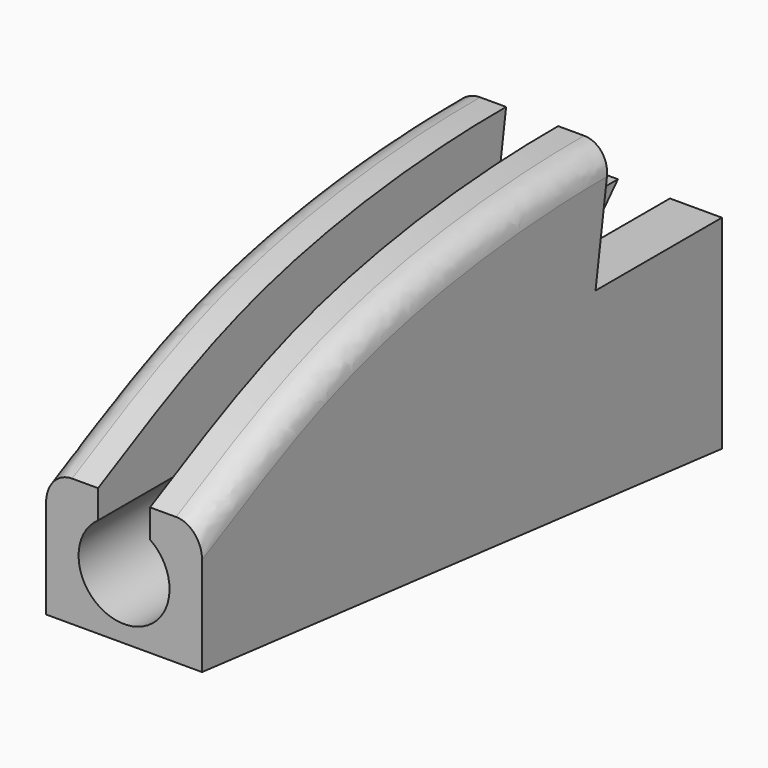
from build123d import *

# Parameters (mm, degrees)
F0_W           = 12
F0_H           = 50
F1_DEPTH       = 30
F3_D           = 7
F3_CSINK_D     = 12
F3_CSINK_ANGLE = 90
F4_W           = 4
F4_H           = 17.1277186767
F5_DEPTH       = 50
F11_DEPTH      = 12.5
F12_R          = 2
F15_DEPTH      = 12.5


# Not quite as in the source:
# - two fillets or chamfers of one size are made in one step
# - the dataset's text gives a spline's control points without its knots; the knots are read off the source's solid


with BuildPart() as f1:
    # F0 (on Top) → F1 (new body)
    with BuildSketch(Plane.XY):
        with Locations((0, -25)):
            Rectangle(F0_W, F0_H)
    extrude(amount=F1_DEPTH)

    # F3 (through all)
    with Locations(Plane(origin=(0, 0, 0), x_dir=(1, 0, 0), z_dir=(0, 1, 0))):
        with Locations((0, -10)):
            CounterSinkHole(F3_D / 2, F3_CSINK_D / 2, counter_sink_angle=F3_CSINK_ANGLE)

    # F4 (on Front) → F5 (cut)
    with BuildSketch(Plane.XZ):
        with Locations((0, 21.4361406616)):
            Rectangle(F4_W, F4_H)
    extrude(amount=F5_DEPTH, mode=Mode.SUBTRACT)

    # F10 (on Right) → F11 (cut, symmetric)
    with BuildSketch(Plane.YZ):
        with BuildLine():
            Line((-12.1560385451, 15.6568542495), (0, 15.6568542495))
            Line((0, 15.6568542495), (0, 30))
            Line((0, 30), (-50, 30))
            Line((-50, 30), (-50, 15.0572415441))
            add(Edge.make_bspline(
                [(-10.7545843348, 24.9280158802), (-18.8047000422, 24.9610823092), (-34.6615045914, 23.1331099195), (-44.5054902356, 17.945709156), (-50, 15.0572415441)],
                knots=[0, 0, 0, 0, 0.5383520225, 1, 1, 1, 1], degree=3))
            Line((-10.7545843348, 24.9280158802), (-12.1560385451, 15.6568542495))
        make_face()
    extrude(amount=F11_DEPTH, both=True, mode=Mode.SUBTRACT)

    # F12
    f12_edges = [f1.edges().sort_by_distance(p)[0] for p in [
        (-6, -31.098721, 22.804231),
        (6, -31.098721, 22.804231),
    ]]
    fillet(f12_edges, radius=F12_R)

    # F14 (on Right) → F15 (cut, symmetric)
    with BuildSketch(Plane.YZ):
        Polygon((0, 0), (-50, 5.1978901029), (-50, 0), align=None)
    extrude(amount=F15_DEPTH, both=True, mode=Mode.SUBTRACT)


solid = f1.part
